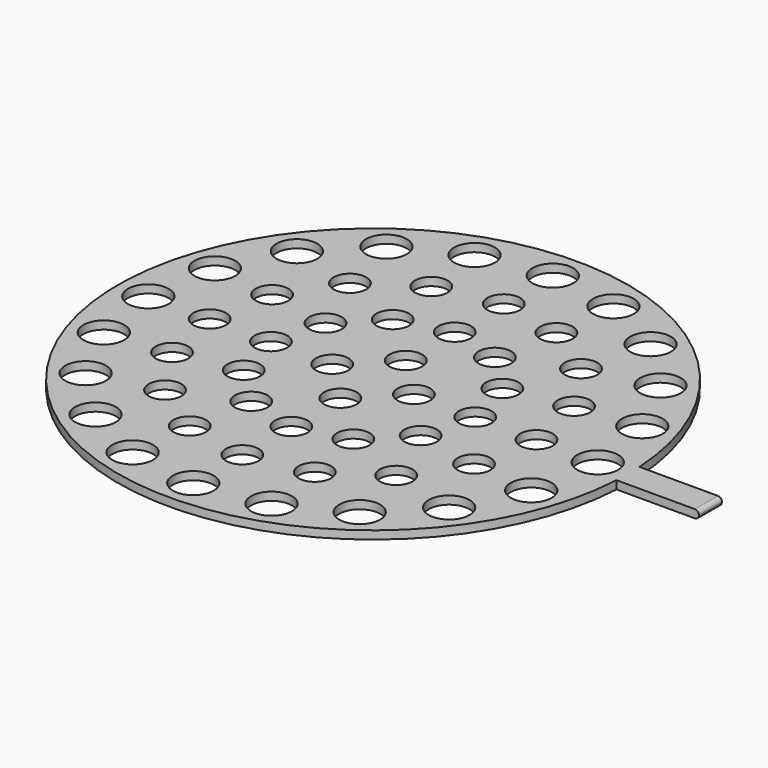
from build123d import *

# Parameters (mm, degrees)
F1_DEPTH         = 2.54
F4_R             = 5.08
F5_DEPTH         = 25.4
F5_COPIES_COUNT  = 16
F6_R             = 6.35
F8_DEPTH         = 25.4
F8_COPIES_COUNT  = 20
F3_R             = 5.08
F9_DEPTH         = 25.4
F9_COPIES_COUNT  = 12
F2_R             = 5.08
F10_DEPTH        = 25.4
F10_COPIES_COUNT = 4
F11_R            = 1.26999


# Not quite as in the source:
# - a fillet or chamfer is up to 0.001 mm smaller than in the source, because OpenCascade refuses the exact size
# - a pattern or mirror of a feature is missing from the dataset's text; its kind, count and spacing are read off the source's solid


with BuildPart() as f1:
    # F0 (on Top) → F1 (new body)
    with BuildSketch(Plane.XY):
        with BuildLine():
            ThreePointArc((79.2488887438, -4.4726119748), (79.343465922, -2.2371947795), (79.375, 0))
            ThreePointArc((79.375, 0), (79.343465922, 2.2371947795), (79.2488887438, 4.4726119748))
            Line((79.2488887438, 4.4726119748), (79.2488887438, -4.4726119748))
        make_face()
        with BuildLine():
            ThreePointArc((79.2488887438, 4.4726119748), (79.343465922, 2.2371947795), (79.375, 0))
            ThreePointArc((79.375, 0), (79.343465922, -2.2371947795), (79.2488887438, -4.4726119748))
            Line((79.2488887438, -4.4726119748), (104.8729870915, -4.4726119748))
            Line((104.8729870915, -4.4726119748), (104.8729870915, 4.4726119748))
            Line((104.8729870915, 4.4726119748), (79.2488887438, 4.4726119748))
        make_face()
        with BuildLine():
            Line((79.2488887438, -4.4726119748), (79.2488887438, 4.4726119748))
            ThreePointArc((79.2488887438, 4.4726119748), (-79.375, 0), (79.2488887438, -4.4726119748))
        make_face()
    extrude(amount=F1_DEPTH)

    # F4 (on Top) → F5 (cut)
    with BuildSketch(Plane.XY):
        with Locations((0, 50.8)):
            Circle(F4_R)
    f5 = extrude(amount=F5_DEPTH, mode=Mode.SUBTRACT)

    # F5_copies: F5 ×16 about axis
    f5_copies_axis = Axis((0, 0, 0), (0, 0, 1))
    for i in range(1, F5_COPIES_COUNT):
        add(f5.rotate(f5_copies_axis, i * 360 / F5_COPIES_COUNT), mode=Mode.SUBTRACT)

    # F6 (on Top) → F8 (cut)
    with BuildSketch(Plane.XY):
        with Locations((0, 69.85)):
            Circle(F6_R)
    f8 = extrude(amount=F8_DEPTH, mode=Mode.SUBTRACT)

    # F8_copies: F8 ×20 about axis
    f8_copies_axis = Axis((0, 0, 0), (0, 0, 1))
    for i in range(1, F8_COPIES_COUNT):
        add(f8.rotate(f8_copies_axis, i * 360 / F8_COPIES_COUNT), mode=Mode.SUBTRACT)

    # F3 (on Top) → F9 (cut)
    with BuildSketch(Plane.XY):
        with Locations((0, 31.75)):
            Circle(F3_R)
    f9 = extrude(amount=F9_DEPTH, mode=Mode.SUBTRACT)

    # F9_copies: F9 ×12 about axis
    f9_copies_axis = Axis((0, 0, 0), (0, 0, 1))
    for i in range(1, F9_COPIES_COUNT):
        add(f9.rotate(f9_copies_axis, i * 360 / F9_COPIES_COUNT), mode=Mode.SUBTRACT)

    # F2 (on Top) → F10 (cut)
    with BuildSketch(Plane.XY):
        with Locations((0, 12.7)):
            Circle(F2_R)
    f10 = extrude(amount=F10_DEPTH, mode=Mode.SUBTRACT)

    # F10_copies: F10 ×4 about axis
    f10_copies_axis = Axis((0, 0, 0), (0, 0, 1))
    for i in range(1, F10_COPIES_COUNT):
        add(f10.rotate(f10_copies_axis, i * 360 / F10_COPIES_COUNT), mode=Mode.SUBTRACT)

    # F11 (radius 1.27 in the source; OpenCascade refuses exactly that, so slightly less here)
    f11_edges = [f1.edges().sort_by_distance(p)[0] for p in [
        (104.872987, 0, 0),
        (104.872987, 0, 2.54),
    ]]
    fillet(f11_edges, radius=F11_R)


solid = f1.part
